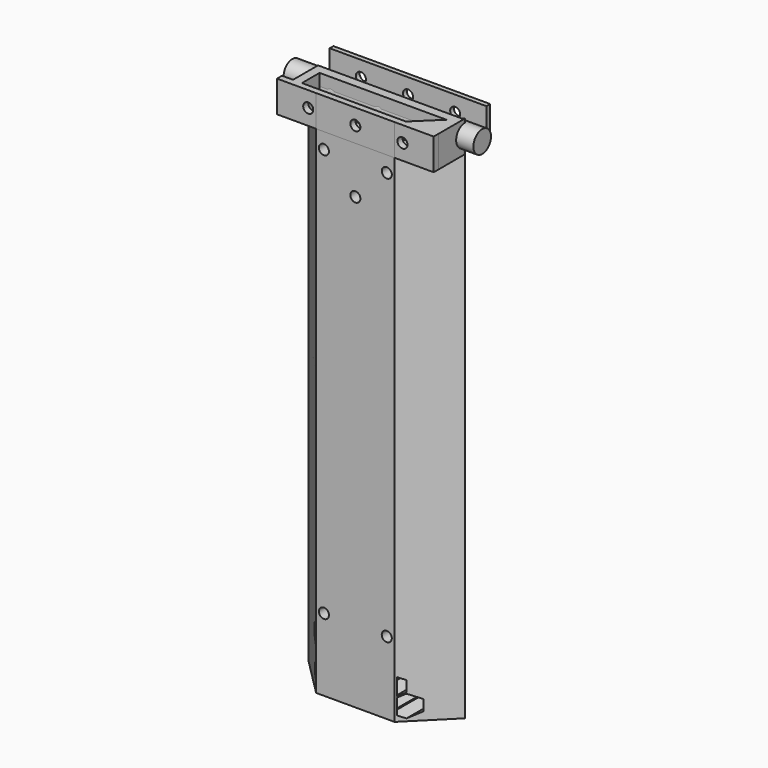
from build123d import *

# Parameters (mm, degrees)
F1_DEPTH       = 138
F3_DEPTH       = 2
F4_W           = 24.9371205636
F4_H           = 0.8
F4_H_2         = 0.2
F5_DEPTH       = 22.4231122666
F7_DEPTH       = 20
F9_DEPTH       = 22
F11_DEPTH      = 80
F13_DEPTH      = 12
F14_D          = 3.2
F14_DEPTH      = 25
F14_TIP        = 0.9613769904
F15_W          = 2.4161204857
F15_H          = 7.042789045
F16_DEPTH      = 10
F15_W_2        = 49.8742333219
F15_H_2        = 1.5
F18_D          = 3.2
F18_DEPTH      = 158.001
F18_ON_F17_D   = 3.2
F18_ON_F17_2_D = 3.2
F19_T1_DEPTH   = 136
F20_T4_DEPTH   = 144.7743645578
F21_R          = 2.15
F21_R_2        = 1
F21_R_3        = 1.25
F22_DEPTH      = 138
F23_R          = 1.6
F24_DEPTH      = 25
F25_R          = 3.5
F26_DEPTH      = 5.2
F26_DEPTH_BACK = 55.2


# Not quite as in the source:
# - a fillet or chamfer that OpenCascade refuses, or shapes differently, is made with other operations: its cross-section is extruded or revolved along the edge and cut away or added
# - a feature names something its author has since deleted; it is built from what else it names


with BuildPart() as f1:
    # F0 (on Top) → F1 (new body)
    with BuildSketch(Plane.XY):
        with BuildLine():
            add(Edge.make_bspline(
                [(-23.2964355304, -74.2783747346), (-23.1790083031, -70.6876792931), (-23.3062370846, -67.1578720119), (-20.7972797666, -65.5632504777)],
                knots=[0.0190145986, 0.0190145986, 0.0190145986, 0.0190145986, 0.3210918621, 0.3210918621, 0.3210918621, 0.3210918621], degree=3))
            Line((-20.7972797666, -65.5632504777), (-25.2154800626, -65.5607786753))
            Line((-25.2154800626, -65.5607786753), (-29.6336803585, -65.5583068728))
            add(Edge.make_bspline(
                [(-27.1442776675, -74.2762220242), (-27.257687128, -70.685397439), (-27.1265088616, -67.1557347261), (-29.6336803585, -65.5583068728)],
                knots=[0.0190145986, 0.0190145986, 0.0190145986, 0.0190145986, 0.3210918621, 0.3210918621, 0.3210918621, 0.3210918621], degree=3))
            ThreePointArc((-27.1442776675, -74.2762220242), (-27.1254979872, -74.6151639935), (-27.1192352516, -74.9545680493))
            ThreePointArc((-27.1192352516, -74.9545680493), (-33.9023805796, -83.8314376267), (-44.2494120982, -79.6185036388))
            ThreePointArc((-44.2494120982, -79.6185036388), (-44.5417990233, -79.0812428635), (-44.7978392579, -78.5257407006))
            add(Edge.make_bspline(
                [(-44.7978392579, -78.5257407006), (-45.9267828866, -76.3008171547), (-47.0706874094, -74.2750328231), (-48.330941751, -73.6820460272)],
                knots=[0.0850609532, 0.0850609532, 0.0850609532, 0.0850609532, 0.6096424985, 0.6096424985, 0.6096424985, 0.6096424985], degree=3))
            Line((-48.330941751, -73.6820460272), (-50.1581720945, -75.5124724791))
            Line((-50.1581720945, -75.5124724791), (-37.7076778796, -87.9769055771))
            Line((-37.7076778796, -87.9769055771), (-12.7483718706, -87.9908692883))
            Line((-12.7483718706, -87.9908692883), (-0.2839387726, -75.5403750734))
            Line((-0.2839387726, -75.5403750734), (-2.1091198754, -73.7079052467))
            add(Edge.make_bspline(
                [(-5.6476398533, -78.5476436364), (-4.5162074246, -76.3239846785), (-3.3700369316, -74.2994815502), (-2.1091198754, -73.7079052467)],
                knots=[0.0850609532, 0.0850609532, 0.0850609532, 0.0850609532, 0.6096424985, 0.6096424985, 0.6096424985, 0.6096424985], degree=3))
            ThreePointArc((-5.6476398533, -78.5476436364), (-5.904301489, -79.1028589635), (-6.1972893817, -79.6397922456))
            ThreePointArc((-6.1972893817, -79.6397922456), (-16.5490283504, -83.8411461177), (-23.3222369441, -74.9566923146))
            ThreePointArc((-23.3222369441, -74.9566923146), (-23.3155944471, -74.6172954788), (-23.2964355304, -74.2783747346))
        make_face()
    extrude(amount=F1_DEPTH)

    # F2 (on face) → F3 (join)
    with BuildSketch(Plane.XY.offset(138)):
        Polygon((-25.2154800626, -65.5607786753), (-40.2154777151, -65.5523867899), (-50.1581720945, -75.5124724791), (-37.7076778796, -87.9769055771), (-12.7483718706, -87.9908692883), (-0.2839387726, -75.5403750734), (-10.21548241, -65.5691705606), align=None)
    extrude(amount=-F3_DEPTH)

    # F6 (on face) → F7 (join)
    with BuildSketch(Plane.XY):
        Polygon((-40.2154777151, -65.5523867899), (-50.1581720945, -75.5124724791), (-37.7076778796, -87.9769055771), (-12.7483718706, -87.9908692883), (-0.2839387726, -75.5403750734), (-10.21548241, -65.5691705606), (-25.2154800626, -65.5607786753), align=None)
    extrude(amount=-F7_DEPTH)

    # F8 (on face) → F9 (cut)
    with BuildSketch(Plane(origin=(-0.0366864559, -65.5748651808, 0), x_dir=(-0.9999998435, 0.000559459, 0), z_dir=(0.000559459, 0.9999998435, 0))):
        Polygon((36.1444616791, -10.7416639358), (33.1444616791, -12.4737147434), (33.1444616791, -15.9378163585), (36.1444616791, -17.6698671661), (39.1444616791, -15.9378163585), (39.1444616791, -12.4737147434), align=None)
        Polygon((37.3925881539, -0.3771449236), (34.3925881539, -2.1091957312), (34.3925881539, -5.5732973463), (37.3925881539, -7.3053481539), (40.3925881539, -5.5732973463), (40.3925881539, -2.1091957312), align=None)
        Polygon((32.5444616791, -5.1991013516), (29.5444616791, -6.9311521592), (29.5444616791, -10.3952537743), (32.5444616791, -12.1273045819), (35.5444616791, -10.3952537743), (35.5444616791, -6.9311521592), align=None)
        Polygon((29.5444616791, -12.8717967697), (26.5444616791, -14.6038475773), (26.5444616791, -18.0679491924), (29.5444616791, -19.8), (32.5444616791, -18.0679491924), (32.5444616791, -14.6038475773), align=None)
        Polygon((23.010861814, -13.8477579841), (20.010861814, -15.5798087916), (20.010861814, -19.0439104068), (21.510861814, -19.9099358105), (25.6999546158, -19.7962056138), (26.2554585934, -15.721026808), align=None)
        Polygon((29.8213052593, 0.8497071097), (26.8213052593, -0.8823436979), (26.8213052593, -4.346445313), (29.8213052593, -6.0784961206), (32.8213052593, -4.346445313), (32.8213052593, -0.8823436979), align=None)
        Polygon((25.9444616791, -4.533019759), (22.9444616791, -6.2650705665), (22.9444616791, -9.7291721817), (25.9444616791, -11.4612229892), (28.9444616791, -9.7291721817), (28.9444616791, -6.2650705665), align=None)
        Polygon((13.410861814, -17.5692959107), (13.410861814, -14.4635716654), (13.5959603421, -14.3567049803), (13.5959603421, -13.9983276106), (10.5959603421, -12.266276803), (7.5959603421, -13.9983276106), (7.5959603421, -17.4624292257), (10.5959603421, -19.1944800333), align=None)
        Polygon((13.5959603421, -14.3567049803), (13.410861814, -14.4635716654), (13.410861814, -17.5692959107), (13.5959603421, -17.4624292257), align=None)
        Polygon((14.1959603421, -14.0102948188), (13.5959603421, -14.3567049803), (13.5959603421, -17.4624292257), (13.410861814, -17.5692959107), (13.410861814, -17.9276732805), (16.410861814, -19.6597240881), (19.410861814, -17.9276732805), (19.410861814, -14.4635716654), (16.410861814, -12.7315208578), align=None)
        Polygon((17.1959603421, -1.1811516346), (14.1959603421, -2.9132024421), (14.1959603421, -6.3773040573), (17.1959603421, -8.1093548648), (20.1959603421, -6.3773040573), (20.1959603421, -2.9132024421), align=None)
        Polygon((13.5959603421, -6.7237142188), (10.5959603421, -8.4557650263), (10.5959603421, -11.9198666415), (13.5959603421, -13.6519174491), (16.5959603421, -11.9198666415), (16.5959603421, -8.4557650263), align=None)
    extrude(amount=-F9_DEPTH, mode=Mode.SUBTRACT)

    # F12 (on face) → F13 (join)
    with BuildSketch(Plane.XY.offset(138)):
        Polygon((-40.2154777151, -65.5523867899), (-47.0690520735, -72.4179491096), (-46.7859623175, -72.7005445625), (-39.8935466375, -65.7960729818), align=None)
    extrude(amount=-F13_DEPTH)

    # F14 (one way)
    with BuildSketch(Plane.XY):
        with Locations((-36.3192352516, -74.9545680493), (-14.1222427032, -74.9669863591)):
            Circle(F14_D / 2)
    extrude(amount=-F14_DEPTH, mode=Mode.SUBTRACT)
    with Locations(Plane.XY):
        with Locations((-36.3192352516, -74.9545680493), (-14.1222427032, -74.9669863591)):
            with Locations((0, 0, -(F14_DEPTH + F14_TIP / 2))):  # 118° drill point
                Cone(0, F14_D / 2, F14_TIP, mode=Mode.SUBTRACT)

    # F18 (through all, one way)
    with BuildSketch(Plane.XY.offset(138)):
        with Locations((-36.3192352516, -74.9545680493), (-14.1222427032, -74.9669863591)):
            Circle(F18_D / 2)
    extrude(amount=-F18_DEPTH, mode=Mode.SUBTRACT)

    # F19: fillet of radius 1 on 2 edges, made by hand

    # F19_s2 → F19_t1 (cut)
    with BuildSketch(Plane.XY):
        with BuildLine():
            ThreePointArc((-23.0780558803, -65.5615744766), (-22.2131010154, -66.0601383234), (-22.2098585164, -67.0584881187))
            Line((-22.2098585164, -67.0584881187), (-22.122982803, -67.108123975))
            ThreePointArc((-22.122982803, -67.108123975), (-21.5239119676, -66.2917415801), (-20.7436100326, -65.6476937572))
            Line((-20.7436100326, -65.6476937572), (-20.7972237897, -65.4631949697))
            ThreePointArc((-20.7972237897, -65.4631949697), (-21.9376119584, -65.4625569692), (-23.0779999033, -65.4615189687))
            Line((-23.0779999033, -65.4615189687), (-23.0780558803, -65.5615744766))
        make_face()
        with BuildLine():
            ThreePointArc((-1.5158594852, -74.3029679616), (-2.2123926892, -74.0081092135), (-2.916636855, -74.2840446053))
            Line((-2.916636855, -74.2840446053), (-2.9857075094, -74.2114276206))
            ThreePointArc((-2.9857075094, -74.2114276206), (-2.5951142627, -73.8833141158), (-2.151687256, -73.6171748777))
            Line((-2.151687256, -73.6171748777), (-2.0381127928, -73.6371805976))
            ThreePointArc((-2.0381127928, -73.6371805976), (-1.7416243006, -73.9348530944), (-1.4448524026, -74.2322433126))
            Line((-1.4448524026, -74.2322433126), (-1.5158594852, -74.3029679616))
        make_face()
    extrude(amount=F19_T1_DEPTH, mode=Mode.SUBTRACT)

    # F20: fillet of radius 2 on 1 edges, made by hand


with BuildPart() as f5:
    # F4 (on face) → F5 (new body, through all)
    with BuildSketch(Plane(origin=(-0.0492312684, -87.9979739382, 0), x_dir=(0.9999998435, -0.000559459, 0), z_dir=(-0.000559459, -0.9999998435, 0))):
        with Locations((-37.6473578289, 65.5)):
            Rectangle(F4_W, F4_H)
        with Locations((-37.6473578289, 66)):
            Rectangle(F4_W, F4_H_2)
        with Locations((-12.7102372653, 65.5)):
            Rectangle(F4_W, F4_H)
    extrude(amount=-F5_DEPTH)


with BuildPart() as f5b:
    # F4 (on face) → F5, piece 2 (new body, through all)
    with BuildSketch(Plane(origin=(-0.0492312684, -87.9979739382, 0), x_dir=(0.9999998435, -0.000559459, 0), z_dir=(-0.000559459, -0.9999998435, 0))):
        Polygon((-50.1159181107, 71.2), (-50.1159181107, 70.8), (-50.1159181107, 70.4), (-25.1787975471, 70.6), (-25.1787975471, 71.2), align=None)
        Polygon((-25.1787975471, 70.6), (-50.1159181107, 70.4), (-50.1159181107, 70.2), (-25.1787975471, 70.2), align=None)
        Polygon((-0.2416769836, 71.2), (-25.1787975471, 71.2), (-25.1787975471, 70.6), (-0.2416769836, 70.8), align=None)
    extrude(amount=-F5_DEPTH)


with BuildPart() as f11_tool:
    # F10 (on face) → F11 (new body)
    with BuildSketch(Plane.XY.offset(138)):
        Polygon((-0.2839387726, -75.5403750734), (-0.2783634016, -65.5747299722), (-10.21548241, -65.5691705606), align=None)
        Polygon((-0.2909082141, -87.9978387301), (-0.2839387726, -75.5403750734), (-12.7483718706, -87.9908692883), align=None)
        Polygon((-37.7076778796, -87.9769055771), (-50.1581720945, -75.5124724791), (-50.1651415361, -87.9699361358), align=None)
        Polygon((-50.1581720945, -75.5124724791), (-40.2154777151, -65.5523867899), (-50.1525967235, -65.5468273781), align=None)
    extrude(amount=-F11_DEPTH)


with BuildPart() as f5_1:
    add(f5.part)

    # F11: cut by f11_tool
    add(f11_tool.part, mode=Mode.SUBTRACT)


with BuildPart() as f5b_1:
    add(f5b.part)

    # F11: cut by f11_tool
    add(f11_tool.part, mode=Mode.SUBTRACT)


with BuildPart() as f16:
    # F15 (on face) → F16 (new body)
    with BuildSketch(Plane.XY.offset(138)):
        Polygon((-50.164022618, -85.9699364488), (-50.1651415361, -87.9699361356), (-37.7076778796, -87.9769055771), (-39.7065586483, -85.9757869723), (-43.8364273338, -85.9734764797), (-46.6561019421, -85.9734764797), (-46.6561019421, -85.971898987), align=None)
        Polygon((-39.7065586483, -85.9757869723), (-37.7076778796, -87.9769055771), (-12.7483718706, -87.9908692883), (-10.7472532658, -85.9919885196), (-11.1188102421, -85.9917806487), align=None)
        Polygon((-10.7472532658, -85.9919885196), (-12.7483718706, -87.9908692883), (-0.2909082141, -87.9978387299), (-0.2897892961, -85.9978390431), (-2.7059097818, -85.9964873225), align=None)
        Polygon((-46.6561019421, -78.9536982775), (-46.6561019421, -85.971898987), (-43.8364273338, -85.9734764797), (-43.8364273338, -78.9536982775), align=None)
        Polygon((-43.8364273338, -85.9734764797), (-46.6561019421, -85.971898987), (-46.6561019421, -85.9734764797), align=None)
        Polygon((-3.4507255796, -78.9536982775), (-10.7472532658, -85.9919885196), (-2.7059097818, -85.9964873225), (-2.7059097818, -78.9536982775), align=None)
        Polygon((-46.6561019421, -78.0811533332), (-46.6561019421, -78.9536982775), (-43.8364273338, -78.9536982775), (-3.8224980537, -78.9536982775), (-0.800840986, -76.0389831733), (-46.6561019421, -76.0389831733), align=None)
        with Locations((-1.4978495389, -82.4750928)):
            Rectangle(F15_W, F15_H)
        Polygon((-3.8224980537, -78.9536982775), (-3.4507255796, -78.9536982775), (-0.4290685119, -76.0389831733), (-0.800840986, -76.0389831733), align=None)
        Polygon((-0.4290685119, -76.0389831733), (-3.4507255796, -78.9536982775), (-2.7059097818, -78.9536982775), (-0.2897892961, -78.9536982775), (-0.2897892961, -76.0389831733), align=None)
        Polygon((-0.800840986, -76.0389831733), (-0.4290685119, -76.0389831733), (-0.2839387726, -75.8989898405), (-0.2839387726, -75.5403750734), align=None)
    extrude(amount=F16_DEPTH)

    # F18 on F17 (through all)
    with Locations(Plane(origin=(-0.0492312684, -87.9979739382, 0), x_dir=(0.9999998435, -0.000559459, 0), z_dir=(-0.000559459, -0.9999998435, 0))):
        with Locations((-40.1787975471, 143), (-25.1787975471, 143), (-10.1787975471, 143)):
            Hole(F18_ON_F17_D / 2)

    # F25 (on Right) → F26 (join, two sides)
    with BuildSketch(Plane.YZ) as f26_sk:
        with Locations((-75.5715926824, 143.3267428094)):
            Circle(F25_R)
    extrude(amount=F26_DEPTH)
    extrude(f26_sk.sketch, amount=-F26_DEPTH_BACK)


with BuildPart() as f16b:
    # F15 (on face) → F16, piece 2 (new body)
    with BuildSketch(Plane.XY.offset(138)):
        with Locations((-25.2154800626, -66.2968273779)):
            Rectangle(F15_W_2, F15_H_2)
    extrude(amount=F16_DEPTH)

    # F18 on F17#2 (through all)
    with Locations(Plane(origin=(-0.0492312684, -87.9979739382, 0), x_dir=(0.9999998435, -0.000559459, 0), z_dir=(-0.000559459, -0.9999998435, 0))):
        with Locations((-40.1787975471, 143), (-25.1787975471, 143), (-10.1787975471, 143)):
            Hole(F18_ON_F17_2_D / 2)


with BuildPart() as f20_tool2:
    # F20_s3 → F20_t4 (new body)
    with BuildSketch(Plane.XY.offset(-8.7743645578)):
        with BuildLine():
            ThreePointArc((-27.7426735927, -68.1692945641), (-27.4521882278, -66.3802051662), (-25.8358535023, -65.5600316016))
            Line((-25.8358535023, -65.5600316016), (-25.8357415795, -65.3599761093))
            ThreePointArc((-25.8357415795, -65.3599761093), (-27.7346551195, -65.3593137449), (-29.6335684357, -65.3582513806))
            Line((-29.6335684357, -65.3582513806), (-29.7411788943, -65.7270263955))
            ThreePointArc((-29.7411788943, -65.7270263955), (-28.6125708149, -66.8110591394), (-27.9332436789, -68.230165368))
            Line((-27.9332436789, -68.230165368), (-27.7426735927, -68.1692945641))
        make_face()
    extrude(amount=F20_T4_DEPTH)

    split(bisect_by=Plane.XY, keep=Keep.TOP)


with BuildPart() as f1_1:
    add(f1.part)

    # F20_t1: cut F20_tool2
    add(f20_tool2.part, mode=Mode.SUBTRACT)

    # F21 (on face) → F22 (cut)
    with BuildSketch(Plane.XY.offset(138)):
        with Locations((-25.2252433966, -83.0121595563)):
            Circle(F21_R)
        with Locations((-25.2168928145, -68.0859889488)):
            Circle(F21_R_2)
        with Locations((-29.5243784785, -84.1509178281)):
            Circle(F21_R_3)
        with Locations((-20.9273851829, -84.1557274943)):
            Circle(F21_R_3)
    extrude(amount=-F22_DEPTH, mode=Mode.SUBTRACT)

    # F23 (on face) → F24 (cut)
    with BuildSketch(Plane(origin=(-0.0492312684, -87.9979739382, 0), x_dir=(0.9999998435, -0.000559459, 0), z_dir=(-0.000559459, -0.9999998435, 0))):
        with Locations((-25.1787975471, 143)):
            Circle(F23_R)
        with Locations((-25.1787975471, 123)):
            Circle(F23_R)
        with Locations((-15.1671273634, 132.978707552)):
            Circle(F23_R)
        with Locations((-35.1904677309, 132.978707552)):
            Circle(F23_R)
        with Locations((-35.1787975471, 3.113188548)):
            Circle(F23_R)
        with Locations((-15.1787975471, 3.113188548)):
            Circle(F23_R)
    extrude(amount=-F24_DEPTH, mode=Mode.SUBTRACT)


solid = Compound([f5_1.part, f5b_1.part, f16.part, f16b.part, f1_1.part])
